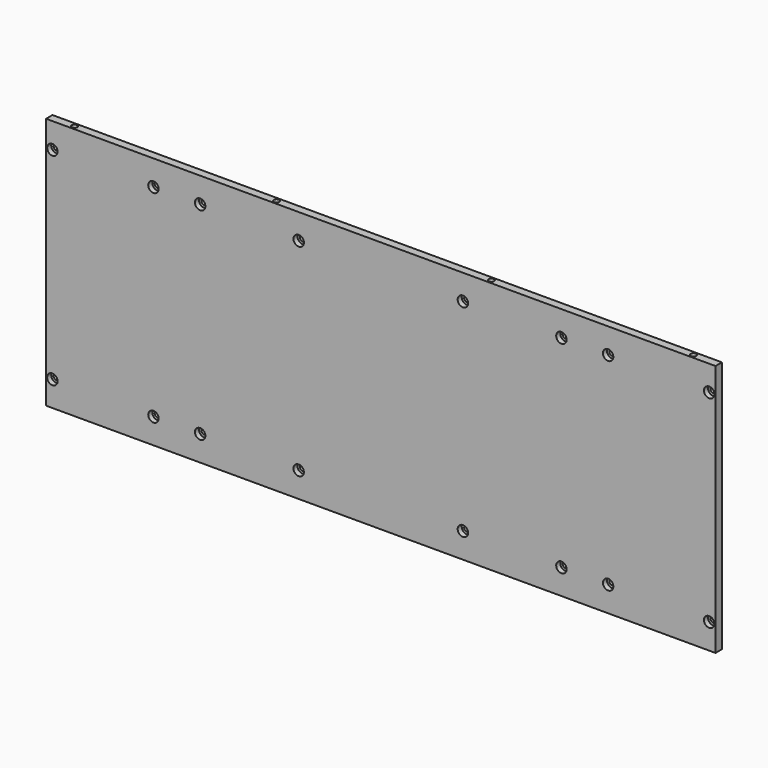
from build123d import *

# Parameters (mm, degrees)
F0_W           = 530
F0_H           = 200
F1_DEPTH       = 3.175
F3_D           = 4.4
F3_DEPTH       = 12
F3_TIP         = 1.3218933619
F5_D           = 4.4
F5_DEPTH       = 10
F5_CBORE_D     = 8.25
F5_CBORE_DEPTH = 4
F5_TIP         = 1.3218933619


# Not quite as in the source:
# - a feature names something its author has since deleted; it is built from what else it names


with BuildPart() as f1:
    # F0 (on Front) → F1 (new body, symmetric)
    with BuildSketch(Plane.XZ):
        Rectangle(F0_W, F0_H)
    extrude(amount=F1_DEPTH, both=True)

    # F3
    with Locations(Plane.XY.offset(100)):
        with Locations((-245, 0), (245, 0), (-85, 0), (85, 0)):
            Hole(F3_D / 2, depth=F3_DEPTH)
            with Locations((0, 0, -(F3_DEPTH + F3_TIP / 2))):  # 118° drill point
                Cone(0, F3_D / 2, F3_TIP, mode=Mode.SUBTRACT)

    # F5
    with Locations(Plane.XZ.offset(3.175)):
        with Locations((-260, 80), (-260, -80), (180, -80), (180, 80), (-143, -80), (-143, 80), (143, -80), (143, 80), (65, -80), (65, 80), (-65, 80), (-65, -80), (260, 80), (260, -80), (-180, 80), (-180, -80)):
            CounterBoreHole(F5_D / 2, F5_CBORE_D / 2, F5_CBORE_DEPTH, depth=F5_DEPTH)
            with Locations((0, 0, -(F5_DEPTH + F5_TIP / 2))):  # 118° drill point
                Cone(0, F5_D / 2, F5_TIP, mode=Mode.SUBTRACT)


solid = f1.part
